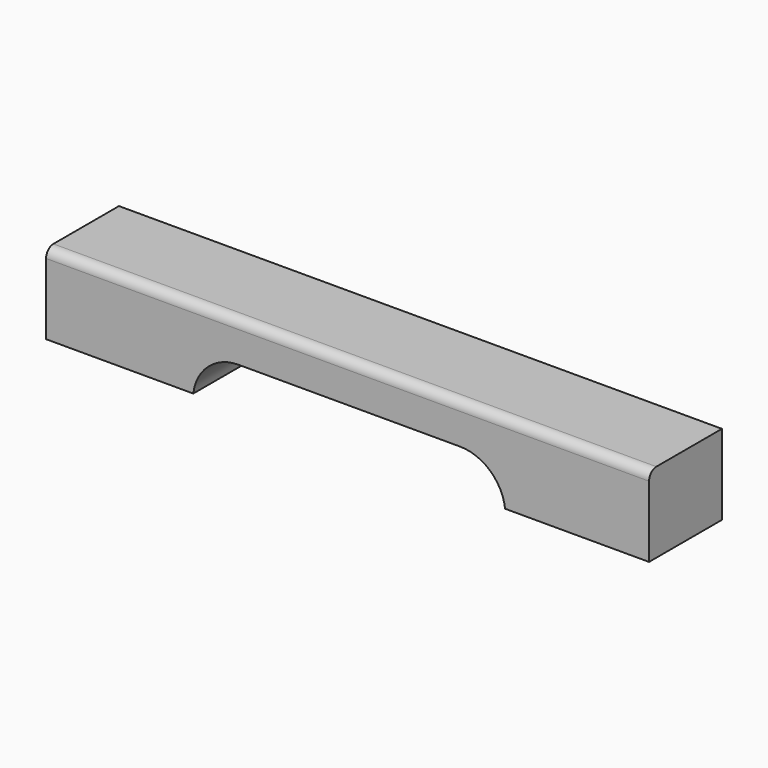
from build123d import *

# Parameters (mm, degrees)
F0_W        = 168.1647002697
F0_H        = 22.3620980978
F1_DEPTH    = 25.4
F2_W        = 86.963314563
F2_H        = 11.1810490489
F3_DEPTH    = 25.4
F4_T1_DEPTH = 25.4
F5_T1_DEPTH = 25.4
F6_R        = 2.54


# Not quite as in the source:
# - a fillet or chamfer that OpenCascade refuses, or shapes differently, is made with other operations: its cross-section is extruded or revolved along the edge and cut away or added


with BuildPart() as f1:
    # F0 (on Front) → F1 (new body)
    with BuildSketch(Plane.XZ):
        Rectangle(F0_W, F0_H)
    extrude(amount=F1_DEPTH)

    # F2 (on face) → F3 (cut)
    with BuildSketch(Plane.XZ.offset(25.4)):
        with Locations((0.4539322108, -5.5905245245)):
            Rectangle(F2_W, F2_H)
    extrude(amount=-F3_DEPTH, mode=Mode.SUBTRACT)

    # F4: fillet of radius 12.7 on 1 edges, made by hand

    # F4_s2 → F4_t1 (join)
    with BuildSketch(Plane.XZ):
        with BuildLine():
            ThreePointArc((-43.0277250707, -11.1810490489), (-38.8450170607, -3.1978771562), (-30.4188873761, 0))
            Line((-30.4188873761, 0), (-43.0277250707, 0))
            Line((-43.0277250707, 0), (-43.0277250707, -11.1810490489))
        make_face()
    extrude(amount=F4_T1_DEPTH)

    # F5: fillet of radius 12.7 on 1 edges, made by hand

    # F5_s2 → F5_t1 (join)
    with BuildSketch(Plane.XZ):
        with BuildLine():
            ThreePointArc((43.9355894923, -11.1810490489), (39.7528814823, -3.1978771562), (31.3267517977, 0))
            Line((31.3267517977, 0), (43.9355894923, 0))
            Line((43.9355894923, 0), (43.9355894923, -11.1810490489))
        make_face()
    extrude(amount=F5_T1_DEPTH)

    # F6
    f6_edges = [f1.edges().sort_by_distance(p)[0] for p in [
        (0, -25.4, 11.181049),
    ]]
    fillet(f6_edges, radius=F6_R)


solid = f1.part
